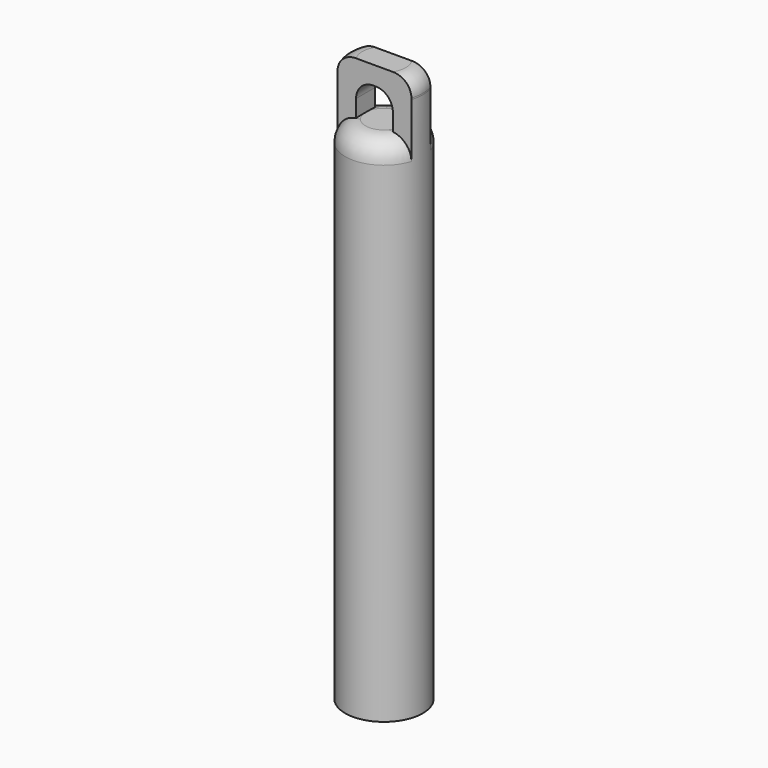
from build123d import *

# Parameters (mm, degrees)
F0_R         = 5.7
F1_DEPTH     = 70
F2_R         = 5.7
F3_DEPTH     = 5
F5_DEPTH     = 5
F6_W         = 5.4
F6_H         = 3.5
F7_DEPTH     = 2.7
F8_R         = 2.5
F9_T4_ANGLE  = 295.1748403761
F9_T9_ANGLE  = 295.1748403761
F9_T15_ANGLE = 295.1748403761
F9_T20_ANGLE = 295.1748403761
F9_T25_ANGLE = 295.1748403761
F9_T31_ANGLE = 295.1748403761


# Not quite as in the source:
# - a fillet or chamfer that OpenCascade refuses, or shapes differently, is made with other operations: its cross-section is extruded or revolved along the edge and cut away or added


with BuildPart() as f1:
    # F0 (on Top) → F1 (new body)
    with BuildSketch(Plane.XY):
        Circle(F0_R)
        Polygon((-2.136195996, -3.7), (-4.272391992, 0), (-2.136195996, 3.7), (2.136195996, 3.7), (4.272391992, 0), (2.136195996, -3.7), align=None, mode=Mode.SUBTRACT)
    extrude(amount=F1_DEPTH)

    # F2 (on face) → F3 (join)
    with BuildSketch(Plane.XY.offset(70)):
        Circle(F2_R)
        Polygon((2.136195996, -3.7), (-2.136195996, -3.7), (-4.272391992, 0), (-2.136195996, 3.7), (2.136195996, 3.7), (4.272391992, 0), align=None, mode=Mode.SUBTRACT)
        Polygon((-4.272391992, 0), (-2.136195996, -3.7), (2.136195996, -3.7), (4.272391992, 0), (2.136195996, 3.7), (-2.136195996, 3.7), align=None)
    extrude(amount=F3_DEPTH)

    # F4 (on face) → F5 (join)
    with BuildSketch(Plane.XY.offset(75)):
        with BuildLine():
            Line((-5.4247119739, -1.75), (-2.7, -1.75))
            Line((-2.7, -1.75), (-2.7, 1.75))
            Line((-2.7, 1.75), (-5.4247119739, 1.75))
            ThreePointArc((-5.4247119739, 1.75), (-5.7, 0), (-5.4247119739, -1.75))
        make_face()
        with BuildLine():
            Line((2.7, -1.75), (5.4247119739, -1.75))
            ThreePointArc((5.4247119739, -1.75), (5.6307574202, -0.8857600546), (5.7, 0))
            ThreePointArc((5.7, 0), (5.6307574202, 0.8857600546), (5.4247119739, 1.75))
            Line((5.4247119739, 1.75), (2.7, 1.75))
            Line((2.7, 1.75), (2.7, -1.75))
        make_face()
    extrude(amount=F5_DEPTH)

    # F6 (on face) → F7 (join)
    with BuildSketch(Plane.XY.offset(80)):
        Rectangle(F6_W, F6_H)
        with BuildLine():
            Line((-2.7, -1.75), (-2.7, 1.75))
            Line((-2.7, 1.75), (-5.4247119739, 1.75))
            ThreePointArc((-5.4247119739, 1.75), (-5.7, 0), (-5.4247119739, -1.75))
            Line((-5.4247119739, -1.75), (-2.7, -1.75))
        make_face()
        with BuildLine():
            Line((5.4247119739, 1.75), (2.7, 1.75))
            Line((2.7, 1.75), (2.7, -1.75))
            Line((2.7, -1.75), (5.4247119739, -1.75))
            ThreePointArc((5.4247119739, -1.75), (5.7, 0), (5.4247119739, 1.75))
        make_face()
    extrude(amount=F7_DEPTH)

    # F8
    f8_edges = [f1.edges().sort_by_distance(p)[0] for p in [
        (-5.7, 0, 82.7),
        (2.7, 0, 80),
        (-2.7, 0, 80),
        (5.7, 0, 82.7),
    ]]
    fillet(f8_edges, radius=F8_R)

    # F9: fillet of radius 3 on 3 edges, made by hand


with BuildPart() as f9_tool2:
    # F9_s3 → F9_t4 (revolve)
    with BuildSketch(Plane(origin=(0, 0, 0), x_dir=(0, 0, 1), z_dir=(0.8442102595, 0.536012162, 0))):
        with BuildLine():
            ThreePointArc((72, -5.7), (74.1213203436, -4.8213203436), (75, -2.7))
            Line((75, -2.7), (75, -5.7))
            Line((75, -5.7), (72, -5.7))
        make_face()
    revolve(axis=Axis((0, 0, 75), (0, 0, 1)), revolution_arc=F9_T4_ANGLE)

    split(bisect_by=Plane.XZ.offset(-1.75), keep=Keep.BOTTOM)


with BuildPart() as f1_1:
    add(f1.part)

    # F9_t1: cut F9_tool2
    add(f9_tool2.part, mode=Mode.SUBTRACT)


with BuildPart() as f9_tool7:
    # F9_s8 → F9_t9 (revolve)
    with BuildSketch(Plane(origin=(0, 0, 0), x_dir=(0, 0, 1), z_dir=(0.8442102595, 0.536012162, 0))):
        with BuildLine():
            ThreePointArc((72, -5.7), (74.1213203436, -4.8213203436), (75, -2.7))
            Line((75, -2.7), (75, -5.7))
            Line((75, -5.7), (72, -5.7))
        make_face()
    revolve(axis=Axis((0, 0, 75), (0, 0, 1)), revolution_arc=F9_T9_ANGLE)

    split(bisect_by=Plane.YZ.offset(-2.7), keep=Keep.TOP)

    split(bisect_by=Plane.YZ.offset(2.7), keep=Keep.BOTTOM)


with BuildPart() as f1_2:
    add(f1_1.part)

    # F9_t6: cut F9_tool7
    add(f9_tool7.part, mode=Mode.SUBTRACT)


with BuildPart() as f9_tool13:
    # F9_s14 → F9_t15 (revolve)
    with BuildSketch(Plane(origin=(0, 0, 0), x_dir=(0, 0, 1), z_dir=(0.8442102595, 0.536012162, 0))):
        with BuildLine():
            ThreePointArc((72, -5.7), (74.1213203436, -4.8213203436), (75, -2.7))
            Line((75, -2.7), (75, -5.7))
            Line((75, -5.7), (72, -5.7))
        make_face()
    revolve(axis=Axis((0, 0, 75), (0, 0, 1)), revolution_arc=F9_T15_ANGLE)

    split(bisect_by=Plane.XZ.offset(1.75), keep=Keep.TOP)


with BuildPart() as f1_3:
    add(f1_2.part)

    # F9_t12: cut F9_tool13
    add(f9_tool13.part, mode=Mode.SUBTRACT)


with BuildPart() as f9_tool18:
    # F9_s19 → F9_t20 (revolve)
    with BuildSketch(Plane(origin=(0, 0, 0), x_dir=(0, 0, 1), z_dir=(-0.8442102595, -0.536012162, 0))):
        with BuildLine():
            ThreePointArc((72, -5.7), (74.1213203436, -4.8213203436), (75, -2.7))
            Line((75, -2.7), (75, -5.7))
            Line((75, -5.7), (72, -5.7))
        make_face()
    revolve(axis=Axis((0, 0, 75), (0, 0, 1)), revolution_arc=F9_T20_ANGLE)

    split(bisect_by=Plane.XZ.offset(1.75), keep=Keep.TOP)


with BuildPart() as f1_4:
    add(f1_3.part)

    # F9_t17: cut F9_tool18
    add(f9_tool18.part, mode=Mode.SUBTRACT)


with BuildPart() as f9_tool23:
    # F9_s24 → F9_t25 (revolve)
    with BuildSketch(Plane(origin=(0, 0, 0), x_dir=(0, 0, 1), z_dir=(-0.8442102595, -0.536012162, 0))):
        with BuildLine():
            ThreePointArc((72, -5.7), (74.1213203436, -4.8213203436), (75, -2.7))
            Line((75, -2.7), (75, -5.7))
            Line((75, -5.7), (72, -5.7))
        make_face()
    revolve(axis=Axis((0, 0, 75), (0, 0, 1)), revolution_arc=F9_T25_ANGLE)

    split(bisect_by=Plane.YZ.offset(-2.7), keep=Keep.TOP)

    split(bisect_by=Plane.YZ.offset(2.7), keep=Keep.BOTTOM)


with BuildPart() as f1_5:
    add(f1_4.part)

    # F9_t22: cut F9_tool23
    add(f9_tool23.part, mode=Mode.SUBTRACT)


with BuildPart() as f9_tool29:
    # F9_s30 → F9_t31 (revolve)
    with BuildSketch(Plane(origin=(0, 0, 0), x_dir=(0, 0, 1), z_dir=(-0.8442102595, -0.536012162, 0))):
        with BuildLine():
            ThreePointArc((72, -5.7), (74.1213203436, -4.8213203436), (75, -2.7))
            Line((75, -2.7), (75, -5.7))
            Line((75, -5.7), (72, -5.7))
        make_face()
    revolve(axis=Axis((0, 0, 75), (0, 0, 1)), revolution_arc=F9_T31_ANGLE)

    split(bisect_by=Plane.XZ.offset(-1.75), keep=Keep.BOTTOM)


with BuildPart() as f1_6:
    add(f1_5.part)

    # F9_t28: cut F9_tool29
    add(f9_tool29.part, mode=Mode.SUBTRACT)


solid = f1_6.part
